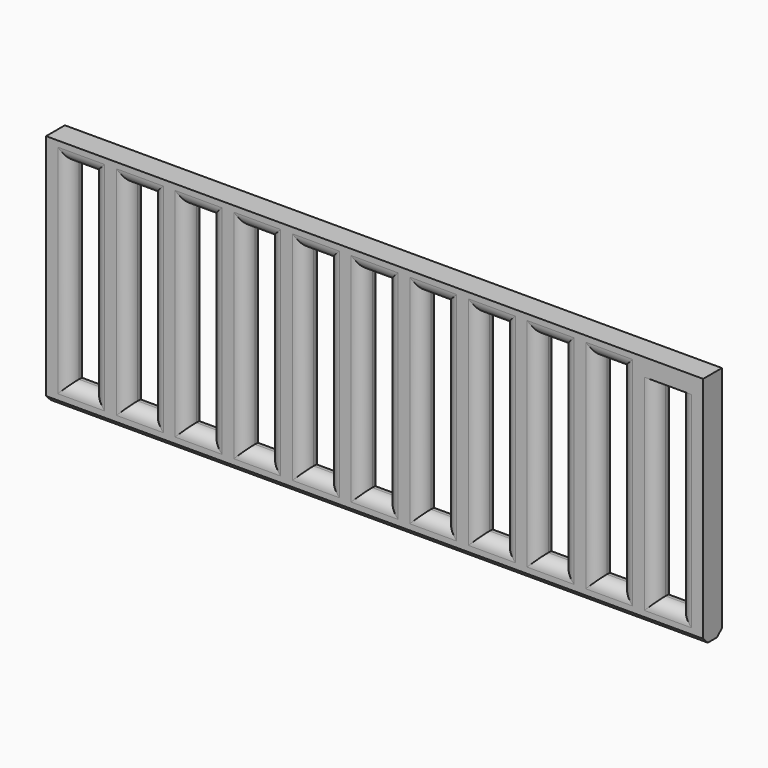
from build123d import *

# Parameters (mm, degrees)
F0_W     = 2844.8
F0_H     = 1016
F1_DEPTH = 101.6
F2_W     = 101.6
F2_H     = 838.2
F3_DEPTH = 307.34
F4_R     = 50.79999
F5_SIZE  = 25.4


# Not quite as in the source:
# - a fillet or chamfer is up to 0.001 mm smaller than in the source, because OpenCascade refuses the exact size


with BuildPart() as f1:
    # F0 (on Front) → F1 (new body)
    with BuildSketch(Plane.XZ):
        with Locations((1422.4, 508)):
            Rectangle(F0_W, F0_H)
    extrude(amount=F1_DEPTH)

    # F2 (on face) → F3 (cut)
    with BuildSketch(Plane.XZ.offset(101.6)):
        with Locations((152.4, 520.7)):
            Rectangle(F2_W, F2_H)
        with Locations((406.4, 520.7)):
            Rectangle(F2_W, F2_H)
        with Locations((660.4, 520.7)):
            Rectangle(F2_W, F2_H)
        with Locations((914.4, 520.7)):
            Rectangle(F2_W, F2_H)
        with Locations((1168.4, 520.7)):
            Rectangle(F2_W, F2_H)
        with Locations((1422.4, 520.7)):
            Rectangle(F2_W, F2_H)
        with Locations((1676.4, 520.7)):
            Rectangle(F2_W, F2_H)
        with Locations((1930.4, 520.7)):
            Rectangle(F2_W, F2_H)
        with Locations((2184.4, 520.7)):
            Rectangle(F2_W, F2_H)
        with Locations((2438.4, 520.7)):
            Rectangle(F2_W, F2_H)
        with Locations((2692.4, 520.7)):
            Rectangle(F2_W, F2_H)
    extrude(amount=-F3_DEPTH, mode=Mode.SUBTRACT)

    # F4 (radius 50.8 in the source; OpenCascade refuses exactly that, so slightly less here)
    f4_edges = [f1.edges().sort_by_distance(p)[0] for p in [
        (101.6, -101.6, 520.7),
        (152.4, -101.6, 939.8),
        (203.2, -101.6, 520.7),
        (152.4, -101.6, 101.6),
        (355.6, -101.6, 520.7),
        (406.4, -101.6, 939.8),
        (457.2, -101.6, 520.7),
        (406.4, -101.6, 101.6),
        (609.6, -101.6, 520.7),
        (660.4, -101.6, 101.6),
        (711.2, -101.6, 520.7),
        (660.4, -101.6, 939.8),
        (863.6, -101.6, 520.7),
        (914.4, -101.6, 939.8),
        (965.2, -101.6, 520.7),
        (914.4, -101.6, 101.6),
        (1117.6, -101.6, 520.7),
        (1168.4, -101.6, 101.6),
        (1219.2, -101.6, 520.7),
        (1168.4, -101.6, 939.8),
        (1422.4, -101.6, 939.8),
        (1371.6, -101.6, 520.7),
        (1473.2, -101.6, 520.7),
        (1422.4, -101.6, 101.6),
        (1676.4, -101.6, 101.6),
        (1625.6, -101.6, 520.7),
        (1727.2, -101.6, 520.7),
        (1676.4, -101.6, 939.8),
        (1879.6, -101.6, 520.7),
        (1930.4, -101.6, 939.8),
        (1981.2, -101.6, 520.7),
        (1930.4, -101.6, 101.6),
        (2184.4, -101.6, 101.6),
        (2133.6, -101.6, 520.7),
        (2235.2, -101.6, 520.7),
        (2184.4, -101.6, 939.8),
        (2438.4, -101.6, 939.8),
        (2387.6, -101.6, 520.7),
        (2489.2, -101.6, 520.7),
        (2438.4, -101.6, 101.6),
        (2641.6, -101.6, 520.7),
        (2692.4, -101.6, 101.6),
        (2743.2, -101.6, 520.7),
        (152.4, 0, 101.6),
        (101.6, 0, 520.7),
        (203.2, 0, 520.7),
        (355.6, 0, 520.7),
        (406.4, 0, 101.6),
        (457.2, 0, 520.7),
        (609.6, 0, 520.7),
        (660.4, 0, 101.6),
        (711.2, 0, 520.7),
        (863.6, 0, 520.7),
        (914.4, 0, 101.6),
        (965.2, 0, 520.7),
        (1117.6, 0, 520.7),
        (1168.4, 0, 101.6),
        (1219.2, 0, 520.7),
        (1422.4, 0, 101.6),
        (1473.2, 0, 520.7),
        (1371.6, 0, 520.7),
        (1625.6, 0, 520.7),
        (1676.4, 0, 101.6),
        (1727.2, 0, 520.7),
        (1879.6, 0, 520.7),
        (1930.4, 0, 101.6),
        (1981.2, 0, 520.7),
        (2133.6, 0, 520.7),
        (2184.4, 0, 101.6),
        (2235.2, 0, 520.7),
        (2387.6, 0, 520.7),
        (2438.4, 0, 101.6),
        (2489.2, 0, 520.7),
        (2641.6, 0, 520.7),
        (2692.4, 0, 101.6),
        (2743.2, 0, 520.7),
    ]]
    fillet(f4_edges, radius=F4_R)

    # F5
    f5_edges = [f1.edges().sort_by_distance(p)[0] for p in [
        (1422.4, 0, 0),
        (1422.4, -101.6, 0),
    ]]
    chamfer(f5_edges, length=F5_SIZE)


solid = f1.part
